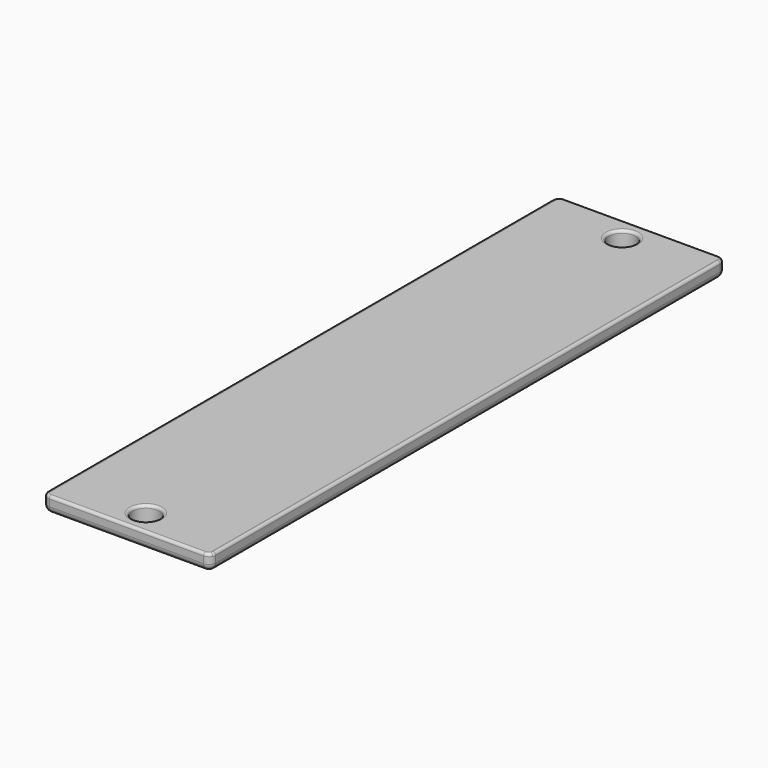
from build123d import *

# Parameters (mm, degrees)
F0_W        = 16.002
F0_H        = 60.96
F0_R        = 1.27
F0_W_2      = 1.905
F1_DEPTH    = 1.524
F2_T1_DEPTH = 72.5997422652
F3_W        = 15.748
F3_H        = 0.254
F4_DEPTH    = 25.4
F5_R        = 0.635
F6_R        = 0.254


# Not quite as in the source:
# - a fillet or chamfer that OpenCascade refuses, or shapes differently, is made with other operations: its cross-section is extruded or revolved along the edge and cut away or added


with BuildPart() as f1:
    # F0 (on Top) → F1 (new body)
    with BuildSketch(Plane.XY):
        Rectangle(F0_W, F0_H)
        with Locations((0, -27.94)):
            Circle(F0_R, mode=Mode.SUBTRACT)
        with Locations((0, 27.94)):
            Circle(F0_R, mode=Mode.SUBTRACT)
        with Locations((-8.9535, 0)):
            Rectangle(F0_W_2, F0_H)
        with Locations((8.9535, 0)):
            Rectangle(F0_W_2, F0_H)
    extrude(amount=F1_DEPTH)

    # F2: fillet of radius 2.54 on 2 edges, made by hand

    # F2_s2 → F2_t1 (cut)
    with BuildSketch(Plane.XZ.offset(-36.2998711326)):
        with BuildLine():
            ThreePointArc((-9.906, 0), (-8.969266843, 1.1091164674), (-7.578051547, 1.524))
            Line((-7.578051547, 1.524), (-9.906, 1.524))
            Line((-9.906, 1.524), (-9.906, 0))
        make_face()
        with BuildLine():
            ThreePointArc((9.906, 0), (8.969266843, 1.1091164674), (7.578051547, 1.524))
            Line((7.578051547, 1.524), (9.906, 1.524))
            Line((9.906, 1.524), (9.906, 0))
        make_face()
    extrude(amount=F2_T1_DEPTH, mode=Mode.SUBTRACT)

    # F3 (on Top) → F4 (cut)
    with BuildSketch(Plane.XY):
        with Locations((0, 30.353)):
            Rectangle(F3_W, F3_H)
        Polygon((11.6183462764, 30.48), (7.874, 30.48), (7.874, 30.226), (7.874, -30.226), (7.874, -30.48), (11.6183462764, -30.48), align=None)
        Polygon((-7.874, 30.226), (-7.874, 30.48), (-11.6183462764, 30.48), (-11.6183462764, -30.48), (-7.874, -30.48), (-7.874, -30.226), align=None)
        with Locations((0, -30.353)):
            Rectangle(F3_W, F3_H)
    extrude(amount=F4_DEPTH, mode=Mode.SUBTRACT)

    # F5
    f5_edges = [f1.edges().sort_by_distance(p)[0] for p in [
        (-7.874, 30.226, 0.75335),
        (7.874, 30.226, 0.75335),
        (-7.874, -30.226, 0.75335),
        (7.874, -30.226, 0.75335),
        (0, -30.226, 0),
        (-7.874, 0, 0),
        (0, 30.226, 0),
        (7.874, 0, 0),
    ]]
    fillet(f5_edges, radius=F5_R)

    # F6
    f6_edges = [f1.edges().sort_by_distance(p)[0] for p in [
        (0, -30.226, 1.524),
        (-1.27, -27.94, 1.524),
        (-1.27, 27.94, 1.524),
        (7.874, 0, 1.5067),
        (-7.874, 0, 1.5067),
        (0, 30.226, 1.524),
        (7.415478, 30.200984, 1.524),
        (7.415478, -30.200984, 1.524),
        (-7.415478, 30.200984, 1.524),
        (-7.415478, -30.200984, 1.524),
        (7.798093, -29.892064, 1.514451),
        (-7.798115, -29.892025, 1.514449),
        (7.798115, 29.892025, 1.514449),
        (-7.798115, 29.892025, 1.514449),
    ]]
    fillet(f6_edges, radius=F6_R)


solid = f1.part
